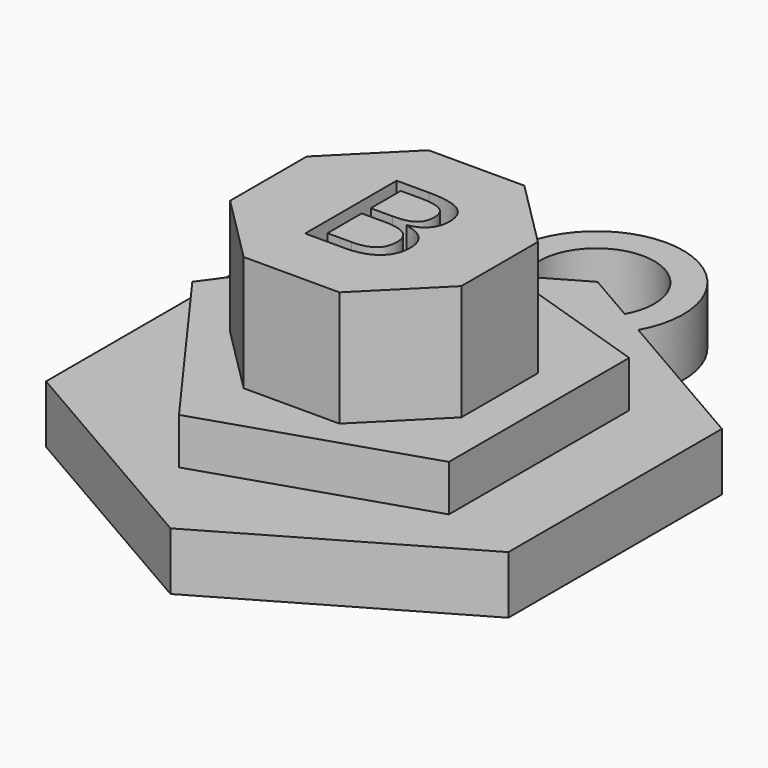
from build123d import *

# Parameters (mm, degrees)
F1_DEPTH     = 3.175
F3_DEPTH     = 2.54
F5_DEPTH     = 6.35
F6_TEXT_SIZE = 8.8045878025
F7_DEPTH     = 12.7
F8_R         = 4.7625
F8_R_2       = 3.175
F9_DEPTH     = 3.175


# Not quite as in the source:
# - Text() gives the source's letters only with a copy of the font that has no kerning and outlines rounded to 1/6400 em; it was checked with that copy


with BuildPart() as f1:
    # F0 (on Top) → F1 (new body)
    with BuildSketch(Plane.XY):
        Polygon((12.7, -7.3323484187), (12.7, 7.3323484187), (0, 14.6646968374), (-12.7, 7.3323484187), (-12.7, -7.3323484187), (0, -14.6646968374), align=None)
    extrude(amount=F1_DEPTH)

    # F2 (on face) → F3 (join)
    with BuildSketch(Plane.XY.offset(3.175)):
        Polygon((8.5194189943, -6.1897202132), (8.5194189943, 6.1897202132), (-3.2541284914, 10.0151776859), (-10.5305810057, 0), (-3.2541284914, -10.0151776859), align=None)
    extrude(amount=F3_DEPTH)

    # F4 (on face) → F5 (join)
    with BuildSketch(Plane.XY.offset(5.715)):
        Polygon((6.35, -2.6302561211), (6.35, 2.6302561211), (2.6302561211, 6.35), (-2.6302561211, 6.35), (-6.35, 2.6302561211), (-6.35, -2.6302561211), (-2.6302561211, -6.35), (2.6302561211, -6.35), align=None)
    extrude(amount=F5_DEPTH)

    # F6 (on face) → F7 (cut)
    with BuildSketch(Plane.XY.offset(12.065)):
        with Locations((-2.7985700872, -2.9995695222)):
            Text('B', F6_TEXT_SIZE, font='Open Sans', text_align=(TextAlign.LEFT, TextAlign.BOTTOM))
    extrude(amount=-F7_DEPTH, mode=Mode.SUBTRACT)

    # F8 (on Top) → F9 (join, through all)
    with BuildSketch(Plane.XY):
        with Locations((0, 14.5934186876)):
            Circle(F8_R)
        with Locations((0, 14.5934186876)):
            Circle(F8_R_2, mode=Mode.SUBTRACT)
    extrude(amount=F9_DEPTH)


solid = f1.part
